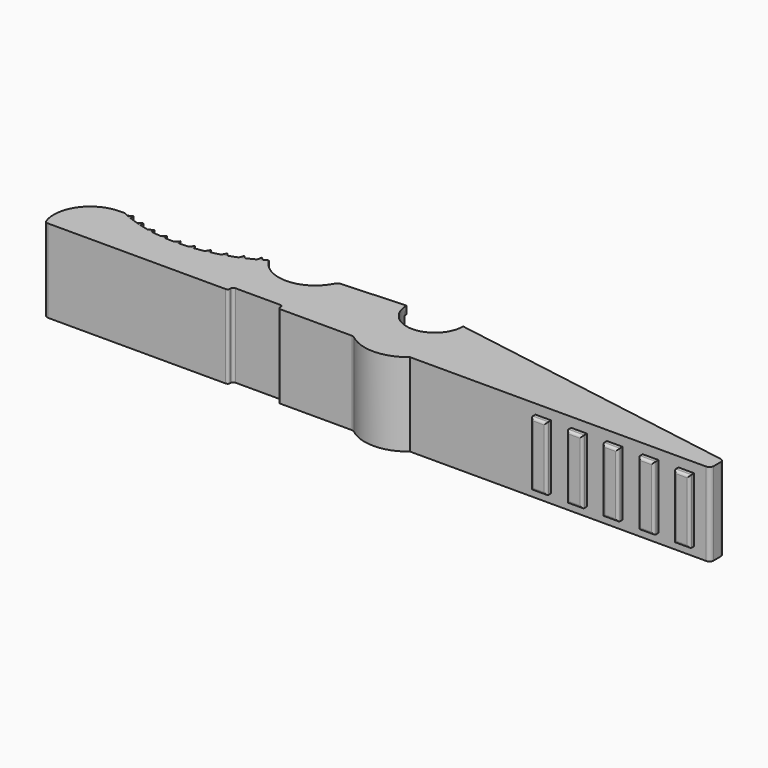
from build123d import *

# Parameters (mm, degrees)
F1_DEPTH     = 10
F2_R         = 0.5
F3_W         = 6.25
F3_H         = 4
F3_W_2       = 5.25
F3_H_2       = 3
F4_DEPTH     = 5.8
F5_R         = 0.5
F6_W         = 1.8886439502
F6_H         = 7.7316380339
F7_DEPTH     = 0.7
F8_R         = 0.3
F9_R         = 0.3
F11_DEPTH    = 6
F12_T1_DEPTH = 7.25
F12_T6_DEPTH = 8.1158070216
F12_S8_R     = 3.4
F12_T9_DEPTH = 6


# Not quite as in the source:
# - a fillet or chamfer that OpenCascade refuses, or shapes differently, is made with other operations: its cross-section is extruded or revolved along the edge and cut away or added


with BuildPart() as f1:
    # F0 (on Top) → F1 (new body)
    with BuildSketch(Plane.XY):
        Polygon((-36.5733099595, 5.6135643101), (-37.0890857119, 5.3072353949), (-36.526321213, 5.1404358199), align=None)
    extrude(amount=F1_DEPTH)


with BuildPart() as f1b:
    # F0 (on Top) → F1, piece 2 (new body)
    with BuildSketch(Plane.XY):
        Polygon((-38.1695665419, 6.1620304579), (-38.7130914025, 5.908174678), (-38.1695665419, 5.6865743499), align=None)
    extrude(amount=F1_DEPTH)


with BuildPart() as f1c:
    # F0 (on Top) → F1, piece 3 (new body)
    with BuildSketch(Plane.XY):
        Polygon((-34.9306636865, 5.2255392929), (-35.4136403219, 4.8697365375), (-34.8371462648, 4.7593708658), align=None)
    extrude(amount=F1_DEPTH)


with BuildPart() as f1d:
    # F0 (on Top) → F1, piece 4 (new body)
    with BuildSketch(Plane.XY):
        Polygon((-33.2577110269, 5.0017545954), (-33.7031596757, 4.599961698), (-33.1185805677, 4.5471105303), align=None)
    extrude(amount=F1_DEPTH)


with BuildPart() as f1e:
    # F0 (on Top) → F1, piece 5 (new body)
    with BuildSketch(Plane.XY):
        Polygon((-31.5708320173, 4.9444013147), (-31.9743912499, 4.5005522674), (-31.38745076, 4.5057330744), align=None)
    extrude(amount=F1_DEPTH)


with BuildPart() as f1f:
    # F0 (on Top) → F1, piece 6 (new body)
    with BuildSketch(Plane.XY):
        with BuildLine():
            ThreePointArc((-40.3752162636, 6.1), (-43.6584529632, 3.9297259752), (-43.8752162636, 0))
            Line((-43.8752162636, 0), (-21.8752162636, 0))
            Line((-21.8752162636, 0), (-21.8752162636, 0.7))
            Line((-21.8752162636, 0.7), (-15.8752162636, 0.7))
            Line((-15.8752162636, 0.7), (-15.8752162636, 0))
            Line((-15.8752162636, 0), (-6.8, 0))
            ThreePointArc((-6.8, 0), (-3.4, -1.2497618994), (0, 0))
            Line((0, 0), (36.1247837364, 0))
            Line((36.1247837364, 0), (36.1247837364, 2))
            Line((36.1247837364, 2), (0, 8))
            ThreePointArc((0, 8), (-3.4, 4.6), (-6.8, 8))
            Line((-6.8, 8), (-14.7261911438, 7.551461916))
            ThreePointArc((-14.7261911438, 7.551461916), (-18.5497691722, 4.8617551386), (-22.6523822876, 7.102923832))
            ThreePointArc((-22.6523822876, 7.102923832), (-22.8908634909, 6.9585259595), (-23.1316147431, 6.8179455041))
            ThreePointArc((-23.1316147431, 6.8179455041), (-23.3874476216, 6.6741154308), (-23.6456566068, 6.5345959996))
            ThreePointArc((-23.6456566068, 6.5345959996), (-24.1560410529, 6.2749236757), (-24.6746482529, 6.0320892243))
            ThreePointArc((-24.6746482529, 6.0320892243), (-24.94344324, 5.9142469288), (-25.2141766861, 5.8009290002))
            ThreePointArc((-25.2141766861, 5.8009290002), (-25.7477256198, 5.5929685859), (-26.2877929861, 5.4025762581))
            ThreePointArc((-26.2877929861, 5.4025762581), (-26.566918285, 5.3118755454), (-26.8475254152, 5.225868626))
            ThreePointArc((-26.8475254152, 5.225868626), (-27.3990148089, 5.0716562811), (-27.9552544913, 4.9355702262))
            ThreePointArc((-27.9552544913, 4.9355702262), (-28.2419771598, 4.8728991555), (-28.5297105235, 4.815045347))
            ThreePointArc((-28.5297105235, 4.815045347), (-29.0937406926, 4.7160909792), (-29.6607064961, 4.6356436285))
            ThreePointArc((-29.6607064961, 4.6356436285), (-29.9522192057, 4.6016158181), (-30.2442615785, 4.5724815725))
            ThreePointArc((-30.2442615785, 4.5724815725), (-30.8153100508, 4.5297540533), (-31.38745076, 4.5057330744))
            ThreePointArc((-31.38745076, 4.5057330744), (-31.6808992824, 4.5006816938), (-31.9743912499, 4.5005522674))
            ThreePointArc((-31.9743912499, 4.5005522674), (-32.5468668362, 4.5144699459), (-33.1185805677, 4.5471105303))
            ThreePointArc((-33.1185805677, 4.5471105303), (-33.4110917209, 4.5710850382), (-33.7031596757, 4.599961698))
            ThreePointArc((-33.7031596757, 4.599961698), (-34.2714572137, 4.6703883049), (-34.8371462648, 4.7593708658))
            ThreePointArc((-34.8371462648, 4.7593708658), (-35.1258560445, 4.8121365254), (-35.4136403219, 4.8697365375))
            ThreePointArc((-35.4136403219, 4.8697365375), (-35.9721955571, 4.9959825193), (-36.526321213, 5.1404358199))
            ThreePointArc((-36.526321213, 5.1404358199), (-36.8084028347, 5.2214759977), (-37.0890857119, 5.3072353949))
            ThreePointArc((-37.0890857119, 5.3072353949), (-37.6324297774, 5.4880646654), (-38.1695665419, 5.6865743499))
            ThreePointArc((-38.1695665419, 5.6865743499), (-38.442258118, 5.7950955739), (-38.7130914025, 5.908174678))
            ThreePointArc((-38.7130914025, 5.908174678), (-38.9972034073, 6.0325947083), (-39.2790657176, 6.1620304579))
            Line((-39.2790657176, 6.1620304579), (-39.8353622856, 6.1305499911))
            Line((-39.8353622856, 6.1305499911), (-40.3752162636, 6.1))
        make_face()
    extrude(amount=F1_DEPTH)

    # F2
    f2_edges = [f1f.edges().sort_by_distance(p)[0] for p in [
        (36.124784, 2, 5),
        (-14.726191, 7.551462, 5),
        (-43.875216, 0, 5),
        (36.124784, 0, 5),
        (-6.8, 0, 5),
    ]]
    fillet(f2_edges, radius=F2_R)

    # F3 (on face) → F4 (join)
    with BuildSketch(Plane(origin=(-0.4729762603, 8.3580422241, 0), x_dir=(-0.9984026576, -0.0564989674, 0), z_dir=(-0.0564989674, 0.9984026576, 0))):
        with Locations((9.4621463323, 2)):
            Rectangle(F3_W, F3_H)
        with Locations((9.4621463323, 2)):
            Rectangle(F3_W_2, F3_H_2, mode=Mode.SUBTRACT)
    extrude(amount=F4_DEPTH)

    # F5
    f5_edges = [f1f.edges().sort_by_distance(p)[0] for p in [
        (-12.704662, 10.570499, 0.5),
        (-12.704662, 10.570499, 3.5),
        (-7.463048, 10.867118, 3.5),
        (-7.463048, 10.867118, 0.5),
    ]]
    fillet(f5_edges, radius=F5_R)

    # F6 (on face) → F7 (join)
    with BuildSketch(Plane.XZ):
        with Locations((33.2505684346, 4.9610123388)):
            Rectangle(F6_W, F6_H)
        with Locations((28.9488484346, 4.9610123388)):
            Rectangle(F6_W, F6_H)
        with Locations((24.6471284346, 4.9610123388)):
            Rectangle(F6_W, F6_H)
        with Locations((20.3454084346, 4.9610123388)):
            Rectangle(F6_W, F6_H)
        with Locations((16.0436884346, 4.9610123388)):
            Rectangle(F6_W, F6_H)
    extrude(amount=F7_DEPTH)

    # F8
    f8_edges = [f1f.edges().sort_by_distance(p)[0] for p in [
        (33.250568, -0.7, 1.095193),
        (34.19489, -0.7, 4.961012),
        (33.250568, -0.7, 8.826831),
        (32.306246, -0.7, 4.961012),
        (28.004526, -0.7, 4.961012),
        (28.948848, -0.7, 1.095193),
        (29.89317, -0.7, 4.961012),
        (28.948848, -0.7, 8.826831),
        (23.702806, -0.7, 4.961012),
        (24.647128, -0.7, 1.095193),
        (25.59145, -0.7, 4.961012),
        (24.647128, -0.7, 8.826831),
        (19.401086, -0.7, 4.961012),
        (20.345408, -0.7, 1.095193),
        (21.28973, -0.7, 4.961012),
        (20.345408, -0.7, 8.826831),
        (15.099366, -0.7, 4.961012),
        (16.043688, -0.7, 1.095193),
        (16.98801, -0.7, 4.961012),
        (16.043688, -0.7, 8.826831),
    ]]
    fillet(f8_edges, radius=F8_R)

    # F9
    f9_edges = [f1f.edges().sort_by_distance(p)[0] for p in [
        (-21.875216, 0, 5),
        (-15.875216, 0, 5),
        (-21.875216, 0.7, 5),
        (-15.875216, 0.7, 5),
    ]]
    fillet(f9_edges, radius=F9_R)

    # F10 (on face) → F11 (cut)
    with BuildSketch(Plane(origin=(-0.4729762603, 8.3580422241, 0), x_dir=(-0.9984026576, -0.0564989674, 0), z_dir=(-0.0564989674, 0.9984026576, 0))):
        Polygon((13.0871463323, 9.5), (6.3371463323, 9.5), (6.3371463323, 4), (12.5871463323, 4), (13.0871463323, 4), align=None)
    extrude(amount=-F11_DEPTH, mode=Mode.SUBTRACT)

    # F12: fillet of radius 0.5 on 2 edges, made by hand

    # F12_s2 → F12_t1 (join)
    with BuildSketch(Plane(origin=(-0.4729762603, 8.3580422241, 0), x_dir=(0, 0, 1), z_dir=(0.0564989674, -0.9984026576, 0))):
        with BuildLine():
            ThreePointArc((9.5, 12.5871463323), (9.3535533906, 12.9406997229), (9, 13.0871463323))
            Line((9, 13.0871463323), (9.5, 13.0871463323))
            Line((9.5, 13.0871463323), (9.5, 12.5871463323))
        make_face()
    extrude(amount=F12_T1_DEPTH)


with BuildPart() as f1g:
    # F0 (on Top) → F1, piece 7 (new body)
    with BuildSketch(Plane.XY):
        Polygon((-28.2213351515, 5.3296001652), (-28.5297105235, 4.815045347), (-27.9552544913, 4.9355702262), align=None)
    extrude(amount=F1_DEPTH)


with BuildPart() as f1h:
    # F0 (on Top) → F1, piece 8 (new body)
    with BuildSketch(Plane.XY):
        Polygon((-29.8865430483, 5.0540410021), (-30.2442615785, 4.5724815725), (-29.6607064961, 4.6356436285), align=None)
    extrude(amount=F1_DEPTH)


with BuildPart() as f1i:
    # F0 (on Top) → F1, piece 9 (new body)
    with BuildSketch(Plane.XY):
        Polygon((-26.8475254152, 5.225868626), (-26.2877929861, 5.4025762581), (-26.5915125336, 5.7683807784), align=None)
    extrude(amount=F1_DEPTH)


with BuildPart() as f1j:
    # F0 (on Top) → F1, piece 10 (new body)
    with BuildSketch(Plane.XY):
        Polygon((-25.2141766861, 5.8009290002), (-24.6746482529, 6.0320892243), (-25.0130329411, 6.3660866994), align=None)
    extrude(amount=F1_DEPTH)


with BuildPart() as f1k:
    # F0 (on Top) → F1, piece 11 (new body)
    with BuildSketch(Plane.XY):
        Polygon((-23.6456566068, 6.5345959996), (-23.1316147431, 6.8179455041), (-23.5013514157, 7.1168657334), align=None)
    extrude(amount=F1_DEPTH)


with BuildPart() as f12_tool4:
    # F12_s5 → F12_t6 (new body)
    with BuildSketch(Plane(origin=(-0.521893463, 9.2224662554, 0), x_dir=(0, 0, 1), z_dir=(0.0564989674, -0.9984026576, 0))):
        with BuildLine():
            ThreePointArc((9.5, 6.8371463323), (9.3535533906, 6.4835929417), (9, 6.3371463323))
            Line((9, 6.3371463323), (9.5, 6.3371463323))
            Line((9.5, 6.3371463323), (9.5, 6.8371463323))
        make_face()
    extrude(amount=F12_T6_DEPTH)

    split(bisect_by=Plane(origin=(-0.4729762603, 8.3580422241, 0), x_dir=(0, 0, 1), z_dir=(0.0564989674, -0.9984026576, 0)), keep=Keep.TOP)

    # F12_s8 → F12_t9 (cut, symmetric)
    with BuildSketch(Plane.XY.offset(9.2)):
        with Locations((-3.4, 8)):
            Circle(F12_S8_R)
    extrude(amount=F12_T9_DEPTH, both=True, mode=Mode.SUBTRACT)


with BuildPart() as f1f_1:
    add(f1f.part)

    # F12_t3: union F12_tool4
    add(f12_tool4.part)


solid = Compound([f1.part, f1b.part, f1c.part, f1d.part, f1e.part, f1g.part, f1h.part, f1i.part, f1j.part, f1k.part, f1f_1.part])
